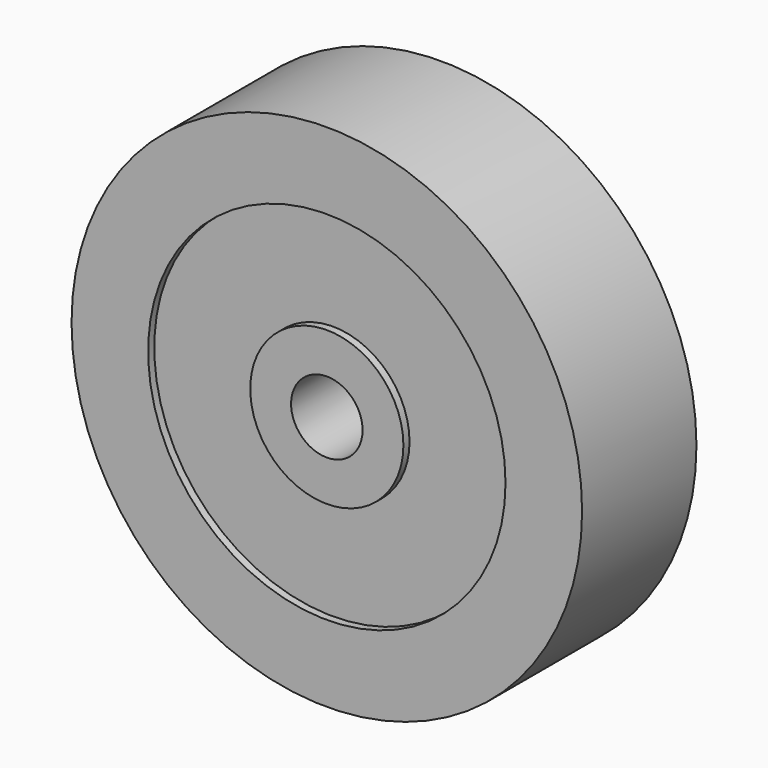
from build123d import *

# Parameters (mm, degrees)
F0_R     = 15
F0_R_2   = 7
F1_DEPTH = 14
F0_R_3   = 50
F0_R_4   = 35
F2_DEPTH = 12.5


with BuildPart() as f1:
    # F0 (on Front) → F1 (new body, symmetric)
    with BuildSketch(Plane.XZ):
        Circle(F0_R)
        Circle(F0_R_2, mode=Mode.SUBTRACT)
    extrude(amount=F1_DEPTH, both=True)


with BuildPart() as f1b:
    # F0 (on Front) → F1, piece 2 (new body, symmetric)
    with BuildSketch(Plane.XZ):
        Circle(F0_R_3)
        Circle(F0_R_4, mode=Mode.SUBTRACT)
    extrude(amount=F1_DEPTH, both=True)

    # F0 (on Front) → F2 (join, symmetric)
    with BuildSketch(Plane.XZ):
        Circle(F0_R_3)
        Circle(F0_R_4, mode=Mode.SUBTRACT)
        Circle(F0_R_4)
        Circle(F0_R, mode=Mode.SUBTRACT)
    extrude(amount=F2_DEPTH, both=True)


solid = Compound([f1.part, f1b.part])
